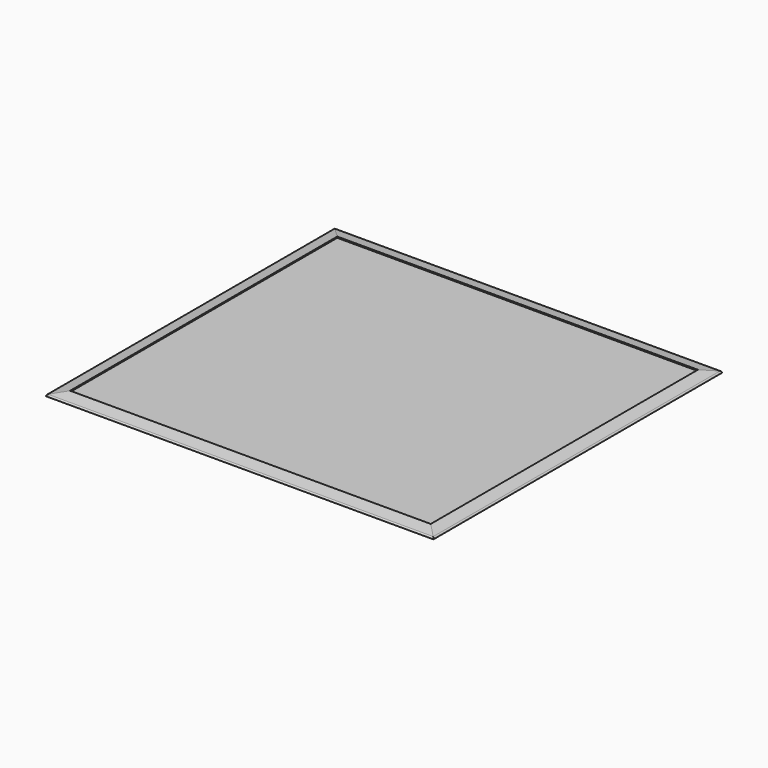
from build123d import *

# Parameters (mm, degrees)
F0_W        = 580
F0_H        = 540
F1_DEPTH    = 7.5
F2_T        = -20
F3_T1_DEPTH = 695.9123277853
F3_T3_DEPTH = 735.9123277853
F4_R        = 2
F5_W        = 540
F5_H        = 500
F6_DEPTH    = 4


# Not quite as in the source:
# - a fillet or chamfer that OpenCascade refuses, or shapes differently, is made with other operations: its cross-section is extruded or revolved along the edge and cut away or added


with BuildPart() as f1:
    # F0 (on Top) → F1 (new body)
    with BuildSketch(Plane.XY):
        with Locations((-1.4553386718, -5.8427717585)):
            Rectangle(F0_W, F0_H)
    extrude(amount=F1_DEPTH)

    # F2
    f2_openings = [f1.faces().sort_by_distance(p)[0] for p in [
        (-1.455339, -5.842772, 7.5),
        (-1.455339, -5.842772, 0),
    ]]
    offset(amount=F2_T, openings=f2_openings)

    # F3: chamfer of 30 x 5.2898094213 on 4 edges, made by hand

    # F3_s2 → F3_t1 (cut)
    with BuildSketch(Plane.XZ.offset(-342.1133921341)):
        Polygon((-291.4553386718, 2.2101905787), (-261.4553386718, 7.5), (-291.4553386718, 7.5), align=None)
        Polygon((288.5446613282, 2.2101905787), (258.5446613282, 7.5), (288.5446613282, 7.5), align=None)
    extrude(amount=F3_T1_DEPTH, mode=Mode.SUBTRACT)

    # F3_s4 → F3_t3 (cut)
    with BuildSketch(Plane.YZ.offset(-369.4115025644)):
        Polygon((-275.8427717585, 2.2101905787), (-245.8427717585, 7.5), (-275.8427717585, 7.5), align=None)
        Polygon((264.1572282415, 2.2101905787), (234.1572282415, 7.5), (264.1572282415, 7.5), align=None)
    extrude(amount=F3_T3_DEPTH, mode=Mode.SUBTRACT)

    # F4
    f4_edges = [f1.edges().sort_by_distance(p)[0] for p in [
        (-291.455339, -5.842772, 2.210191),
        (-1.455339, -275.842772, 2.210191),
        (288.544661, -5.842772, 2.210191),
        (-1.455339, 264.157228, 2.210191),
    ]]
    fillet(f4_edges, radius=F4_R)

    # F5 (on Top) → F6 (join)
    with BuildSketch(Plane.XY):
        with Locations((-1.4553386718, -5.8427717585)):
            Rectangle(F5_W, F5_H)
    extrude(amount=F6_DEPTH)


solid = f1.part
